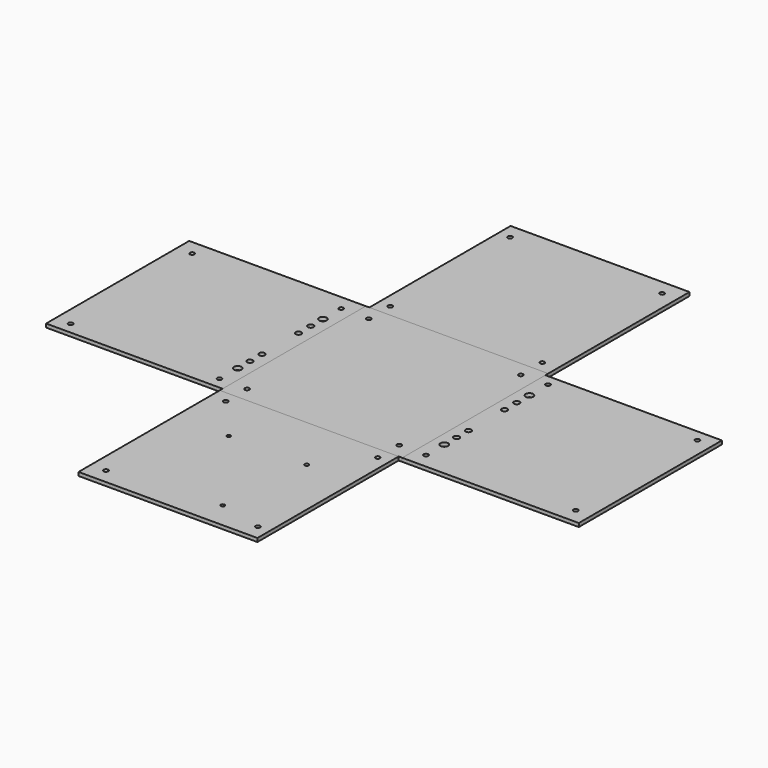
from build123d import *

# Parameters (mm, degrees)
F0_R     = 1.905
F1_DEPTH = 2.9972
F0_W     = 149.4028
F0_H     = 147.4714428186
F2_DEPTH = 2.9972
F0_W_2   = 147.4714428186
F0_H_2   = 149.4028
F0_R_2   = 3.175
F0_R_3   = 2.38125
F3_DEPTH = 2.9972
F0_W_3   = 84.8
F0_H_3   = 90.25
F4_DEPTH = 2.9972
F5_DEPTH = 2.9972
F0_R_4   = 1.5875
F6_DEPTH = 2.9972


# Not quite as in the source:
# - a feature names something its author has since deleted; it is built from what else it names


with BuildPart() as f1:
    # F0 (on Top) → F1 (new body)
    with BuildSketch(Plane.XY):
        Polygon((0, 2.9972), (0, 0), (149.4028, 0), (152.4, 0), (152.4, 149.4028), (152.4, 152.4), (2.9972, 152.4), (0, 152.4), align=None)
        with Locations((12.7, 12.7)):
            Circle(F0_R, mode=Mode.SUBTRACT)
        with Locations((139.7, 12.7)):
            Circle(F0_R, mode=Mode.SUBTRACT)
        with Locations((12.7, 139.7)):
            Circle(F0_R, mode=Mode.SUBTRACT)
        with Locations((139.7, 139.7)):
            Circle(F0_R, mode=Mode.SUBTRACT)
    extrude(amount=F1_DEPTH)


with BuildPart() as f2:
    # F0 (on Top) → F2 (new body)
    with BuildSketch(Plane.XY):
        with Locations((77.6986, 226.1357214093)):
            Rectangle(F0_W, F0_H)
        with Locations((12.7, 162.1028)):
            Circle(F0_R, mode=Mode.SUBTRACT)
        with Locations((12.7, 287.1714428186)):
            Circle(F0_R, mode=Mode.SUBTRACT)
        with Locations((139.7, 162.1028)):
            Circle(F0_R, mode=Mode.SUBTRACT)
        with Locations((139.7, 287.1714428186)):
            Circle(F0_R, mode=Mode.SUBTRACT)
    extrude(amount=F2_DEPTH)


with BuildPart() as f3:
    # F0 (on Top) → F3 (new body)
    with BuildSketch(Plane.XY):
        with Locations((-73.7357214093, 77.6986)):
            Rectangle(F0_W_2, F0_H_2)
        with Locations((-134.7714428186, 12.7)):
            Circle(F0_R, mode=Mode.SUBTRACT)
        with Locations((-10.3772366419, 12.7)):
            Circle(F0_R, mode=Mode.SUBTRACT)
        with Locations((-10.3772366419, 31.75)):
            Circle(F0_R_2, mode=Mode.SUBTRACT)
        with Locations((-10.3772366419, 44.45)):
            Circle(F0_R_3, mode=Mode.SUBTRACT)
        with Locations((-10.3772366419, 57.15)):
            Circle(F0_R_3, mode=Mode.SUBTRACT)
        with Locations((-134.7714428186, 139.7)):
            Circle(F0_R, mode=Mode.SUBTRACT)
        with Locations((-10.3772366419, 95.25)):
            Circle(F0_R_3, mode=Mode.SUBTRACT)
        with Locations((-10.3772366419, 107.95)):
            Circle(F0_R_3, mode=Mode.SUBTRACT)
        with Locations((-10.3772366419, 120.65)):
            Circle(F0_R_2, mode=Mode.SUBTRACT)
        with Locations((-10.3772366419, 139.7)):
            Circle(F0_R, mode=Mode.SUBTRACT)
    extrude(amount=F3_DEPTH)


with BuildPart() as f4:
    # F0 (on Top) → F4 (new body)
    with BuildSketch(Plane.XY):
        with Locations((74.7014, -73.7357214093)):
            Rectangle(F0_W, F0_H)
        with Locations((12.7, -134.7714428186)):
            Circle(F0_R, mode=Mode.SUBTRACT)
        with Locations((75.2196, -86.5296946764)):
            Rectangle(F0_W_3, F0_H_3, mode=Mode.SUBTRACT)
        with Locations((12.7, -9.7028)):
            Circle(F0_R, mode=Mode.SUBTRACT)
        with Locations((139.7, -134.7714428186)):
            Circle(F0_R, mode=Mode.SUBTRACT)
        with Locations((139.7, -9.7028)):
            Circle(F0_R, mode=Mode.SUBTRACT)
    extrude(amount=F4_DEPTH)

    # F0 (on Top) → F6 (join)
    with BuildSketch(Plane.XY):
        with Locations((75.2196, -86.5296946764)):
            Rectangle(F0_W_3, F0_H_3)
        with Locations((44.8646, -46.6086946764)):
            Circle(F0_R_4, mode=Mode.SUBTRACT)
        with Locations((102.9745078107, -125.5666946764)):
            Circle(F0_R_4, mode=Mode.SUBTRACT)
        with Locations((109.8646, -46.6086946764)):
            Circle(F0_R_4, mode=Mode.SUBTRACT)
    extrude(amount=F6_DEPTH)


with BuildPart() as f5:
    # F0 (on Top) → F5 (new body)
    with BuildSketch(Plane.XY):
        with Locations((226.1357214093, 74.7014)):
            Rectangle(F0_W_2, F0_H_2)
        with Locations((162.1028, 12.7)):
            Circle(F0_R, mode=Mode.SUBTRACT)
        with Locations((162.1028, 31.75)):
            Circle(F0_R_2, mode=Mode.SUBTRACT)
        with Locations((162.1028, 44.5710918487)):
            Circle(F0_R_3, mode=Mode.SUBTRACT)
        with Locations((162.1028, 56.9709617438)):
            Circle(F0_R_3, mode=Mode.SUBTRACT)
        with Locations((287.1714428186, 12.7)):
            Circle(F0_R, mode=Mode.SUBTRACT)
        with Locations((162.1028, 94.7086235553)):
            Circle(F0_R_3, mode=Mode.SUBTRACT)
        with Locations((162.1028, 107.4299048555)):
            Circle(F0_R_3, mode=Mode.SUBTRACT)
        with Locations((162.1028, 120.65)):
            Circle(F0_R_2, mode=Mode.SUBTRACT)
        with Locations((162.1028, 140.0506034862)):
            Circle(F0_R, mode=Mode.SUBTRACT)
        with Locations((287.1714428186, 139.7)):
            Circle(F0_R, mode=Mode.SUBTRACT)
    extrude(amount=F5_DEPTH)


solid = Compound([f1.part, f2.part, f3.part, f4.part, f5.part])
